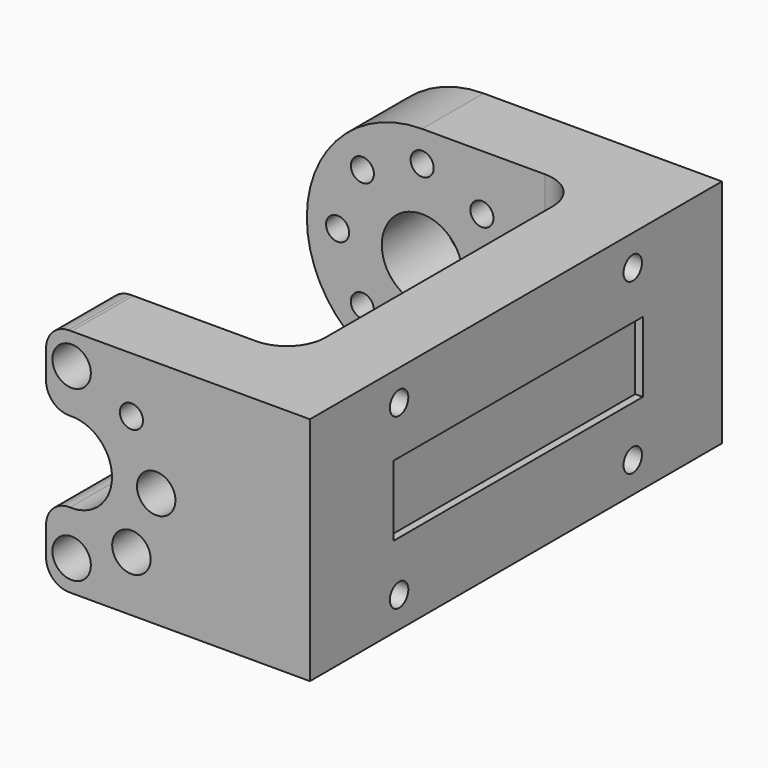
from build123d import *

# Parameters (mm, degrees)
F1_DEPTH  = 30
F2_R      = 14.99999
F3_R      = 5.25
F4_DEPTH  = 100
F5_R      = 2.5
F6_DEPTH  = 7
F7_DEPTH  = 7
F8_R      = 1.5
F9_DEPTH  = 100
F10_R     = 2.5
F10_R_2   = 1.5
F11_DEPTH = 7
F12_W     = 19.7517806664
F12_H     = 36.5692139603
F13_DEPTH = 25
F14_R     = 3
F15_R     = 5
F16_R     = 1.5
F17_DEPTH = 25
F18_W     = 40.5211038888
F18_H     = 9.174589999
F19_DEPTH = 1


# Not quite as in the source:
# - a fillet or chamfer is up to 0.001 mm smaller than in the source, because OpenCascade refuses the exact size


with BuildPart() as f1:
    # F0 (on Top) → F1 (new body)
    with BuildSketch(Plane.XY):
        Polygon((26.5140141845, 39.809118801), (-19.4859858155, 39.809118801), (-19.4859858155, 29.809118801), (16.5140141845, 29.809118801), (16.5140141845, -17.190881199), (-19.4859858155, -17.190881199), (-19.4859858155, -27.190881199), (26.5140141845, -27.190881199), align=None)
    extrude(amount=F1_DEPTH)

    # F2 (radius 15 in the source; OpenCascade refuses exactly that, so slightly less here)
    f2_edges = [f1.edges().sort_by_distance(p)[0] for p in [
        (-19.485986, 34.809119, 30),
        (-19.485986, 34.809119, 0),
        (-19.485986, -22.190881, 30),
        (-19.485986, -22.190881, 0),
    ]]
    fillet(f2_edges, radius=F2_R)

    # F3 (on face) → F4 (cut)
    with BuildSketch(Plane(origin=(0, 39.809118801, 0), x_dir=(-1, 0, 0), z_dir=(0, 1, 0))):
        with Locations((4.4859858155, 15)):
            Circle(F3_R)
    extrude(amount=-F4_DEPTH, mode=Mode.SUBTRACT)

    # F5 (on face) → F6 (cut)
    with BuildSketch(Plane(origin=(0, 39.809118801, 0), x_dir=(-1, 0, 0), z_dir=(0, 1, 0))):
        with Locations((4.4859858155, 26)):
            Circle(F5_R)
    extrude(amount=-F6_DEPTH, mode=Mode.SUBTRACT)

    # F5 (on face) → F7 (cut)
    with BuildSketch(Plane(origin=(0, 39.809118801, 0), x_dir=(-1, 0, 0), z_dir=(0, 1, 0))):
        with Locations((-3.2921887775, 22.7781745931)):
            Circle(F5_R)
        with Locations((-6.5140141845, 15)):
            Circle(F5_R)
        with Locations((-3.2921887775, 7.2218254069)):
            Circle(F5_R)
        with Locations((4.4859858155, 4)):
            Circle(F5_R)
        with Locations((12.2641604086, 7.2218254069)):
            Circle(F5_R)
        with Locations((15.4859858155, 15)):
            Circle(F5_R)
        with Locations((12.2641604086, 22.7781745931)):
            Circle(F5_R)
    extrude(amount=-F7_DEPTH, mode=Mode.SUBTRACT)

    # F8 (on face) → F9 (cut)
    with BuildSketch(Plane(origin=(0, 39.809118801, 0), x_dir=(-1, 0, 0), z_dir=(0, 1, 0))):
        with Locations((4.4859858155, 26)):
            Circle(F8_R)
        with Locations((12.2641604086, 22.7781745931)):
            Circle(F8_R)
        with Locations((15.4859858155, 15)):
            Circle(F8_R)
        with Locations((12.2641604086, 7.2218254069)):
            Circle(F8_R)
        with Locations((4.4859858155, 4)):
            Circle(F8_R)
        with Locations((-3.2921887775, 7.2218254069)):
            Circle(F8_R)
        with Locations((-6.5140141845, 15)):
            Circle(F8_R)
        with Locations((-3.2921887775, 22.7781745931)):
            Circle(F8_R)
    extrude(amount=-F9_DEPTH, mode=Mode.SUBTRACT)

    # F10 (on face) → F11 (cut)
    with BuildSketch(Plane.XZ.offset(27.190881199)):
        with Locations((-4.4859858155, 26)):
            Circle(F10_R)
        with Locations((-4.4859858155, 26)):
            Circle(F10_R_2, mode=Mode.SUBTRACT)
        with Locations((-12.2641604086, 22.7781745931)):
            Circle(F10_R)
        with Locations((-12.2641604086, 22.7781745931)):
            Circle(F10_R_2, mode=Mode.SUBTRACT)
        with Locations((-15.4859858155, 15)):
            Circle(F10_R)
        with Locations((-15.4859858155, 15)):
            Circle(F10_R_2, mode=Mode.SUBTRACT)
        with Locations((-12.2641604086, 7.2218254069)):
            Circle(F10_R)
        with Locations((-12.2641604086, 7.2218254069)):
            Circle(F10_R_2, mode=Mode.SUBTRACT)
        with Locations((-4.4859858155, 4)):
            Circle(F10_R)
        with Locations((-4.4859858155, 4)):
            Circle(F10_R_2, mode=Mode.SUBTRACT)
        with Locations((3.2921887775, 7.2218254069)):
            Circle(F10_R)
        with Locations((3.2921887775, 7.2218254069)):
            Circle(F10_R_2, mode=Mode.SUBTRACT)
        with Locations((6.5140141845, 15)):
            Circle(F10_R)
        with Locations((6.5140141845, 15)):
            Circle(F10_R_2, mode=Mode.SUBTRACT)
        with Locations((-4.4859858155, 26)):
            Circle(F10_R_2)
    extrude(amount=-F11_DEPTH, mode=Mode.SUBTRACT)

    # F12 (on face) → F13 (cut)
    with BuildSketch(Plane.XZ.offset(27.190881199)):
        with Locations((-17.6862510853, 15.8640302252)):
            Rectangle(F12_W, F12_H)
    extrude(amount=-F13_DEPTH, mode=Mode.SUBTRACT)

    # F14
    f14_edges = [f1.edges().sort_by_distance(p)[0] for p in [
        (-7.810361, -22.190881, 29.626982),
        (-7.810361, -22.190881, 0.373018),
        (-7.810361, -22.190881, 10.936623),
        (-7.810361, -22.190881, 19.063377),
    ]]
    fillet(f14_edges, radius=F14_R)

    # F15
    f15_edges = [f1.edges().sort_by_distance(p)[0] for p in [
        (16.514014, 29.809119, 15),
        (16.514014, -17.190881, 15),
    ]]
    fillet(f15_edges, radius=F15_R)

    # F16 (on face) → F17 (cut)
    with BuildSketch(Plane.YZ.offset(26.5140141845)):
        with Locations((-12.690881199, 26)):
            Circle(F16_R)
        with Locations((-12.690881199, 4)):
            Circle(F16_R)
        with Locations((25.309118801, 4)):
            Circle(F16_R)
        with Locations((25.309118801, 26)):
            Circle(F16_R)
    extrude(amount=-F17_DEPTH, mode=Mode.SUBTRACT)

    # F18 (on face) → F19 (cut)
    with BuildSketch(Plane.YZ.offset(26.5140141845)):
        with Locations((6.6909566522, 15.1345017366)):
            Rectangle(F18_W, F18_H)
    extrude(amount=-F19_DEPTH, mode=Mode.SUBTRACT)


solid = f1.part
